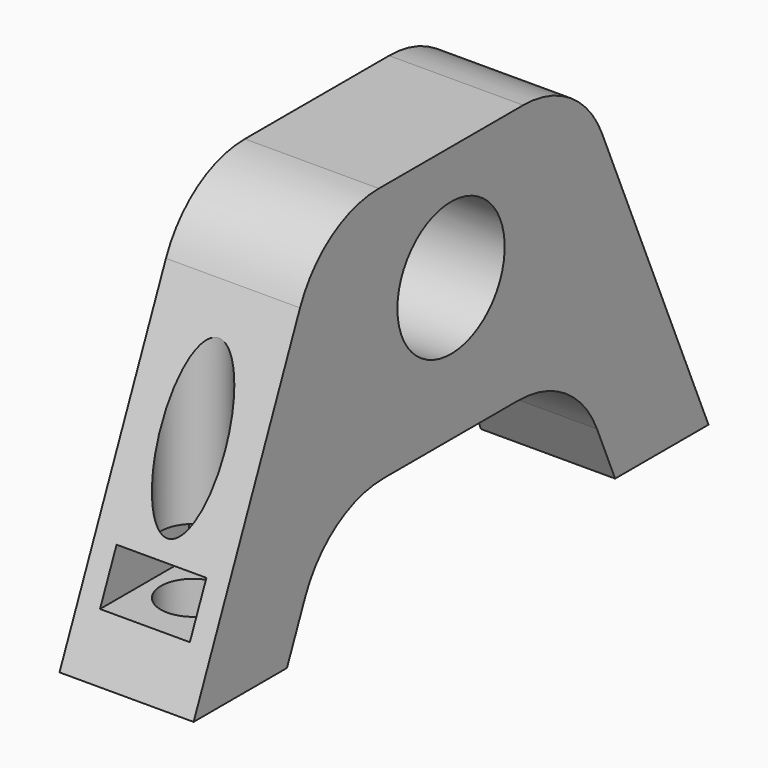
from build123d import *

# Parameters (mm, degrees)
F1_DEPTH  = 25
F2_R      = 5
F3_DEPTH  = 15
F5_DEPTH  = 25
F7_W      = 16.75
F7_H      = 9
F8_DEPTH  = 25
F9_R      = 6
F10_DEPTH = 50
F11_R     = 20
F2_R_2    = 12.5
F12_DEPTH = 25


# Not quite as in the source:
# - a pattern or mirror of a feature is missing from the dataset's text; its kind, count and spacing are read off the source's solid


with BuildPart() as f1:
    # F0 (on Right) → F1 (new body)
    with BuildSketch(Plane.YZ):
        Polygon((-60, -35), (60, -35), (30, 35), (-30, 35), align=None)
    extrude(amount=F1_DEPTH)

    # F2 (on face) → F3 (cut)
    with BuildSketch(Plane(origin=(0, 0, 0), x_dir=(0, -1, 0), z_dir=(-1, 0, 0))):
        with Locations((-30, 13.5)):
            Circle(F2_R)
        with Locations((30, 13.5)):
            Circle(F2_R)
    extrude(amount=-F3_DEPTH, mode=Mode.SUBTRACT)

    # F4 (on face) → F5 (cut)
    with BuildSketch(Plane(origin=(0, 0, 0), x_dir=(0, -1, 0), z_dir=(-1, 0, 0))):
        Polygon((-28.8120768404, -13), (-38.240648269, -35), (38.240648269, -35), (28.8120768404, -13), align=None)
    extrude(amount=-F5_DEPTH, mode=Mode.SUBTRACT)

    # F7 (on offset) → F8 (cut)
    with BuildSketch(Plane.XZ.offset(60)):
        with Locations((12.5, -20.5)):
            Rectangle(F7_W, F7_H)
    f8 = extrude(amount=-F8_DEPTH, mode=Mode.SUBTRACT)

    # F8_copies: F8 across plane
    add(f8.mirror(Plane.ZX), mode=Mode.SUBTRACT)

    # F9 (on face) → F10 (cut, symmetric)
    with BuildSketch(Plane.XY.offset(-25)):
        with Locations((12.5, -44.487604307)):
            Circle(F9_R)
    f10 = extrude(amount=F10_DEPTH, both=True, mode=Mode.SUBTRACT)

    # F10_copies: F10 across plane
    add(f10.mirror(Plane.ZX), mode=Mode.SUBTRACT)

    # F11
    f11_edges = [f1.edges().sort_by_distance(p)[0] for p in [
        (12.5, -28.812077, -13),
        (12.5, 28.812077, -13),
        (12.5, 30, 35),
        (12.5, -30, 35),
    ]]
    fillet(f11_edges, radius=F11_R)

    # F2 (on face) → F12 (cut)
    with BuildSketch(Plane(origin=(0, 0, 0), x_dir=(0, -1, 0), z_dir=(-1, 0, 0))):
        with Locations((0, 13.5)):
            Circle(F2_R_2)
    extrude(amount=-F12_DEPTH, mode=Mode.SUBTRACT)


solid = f1.part
